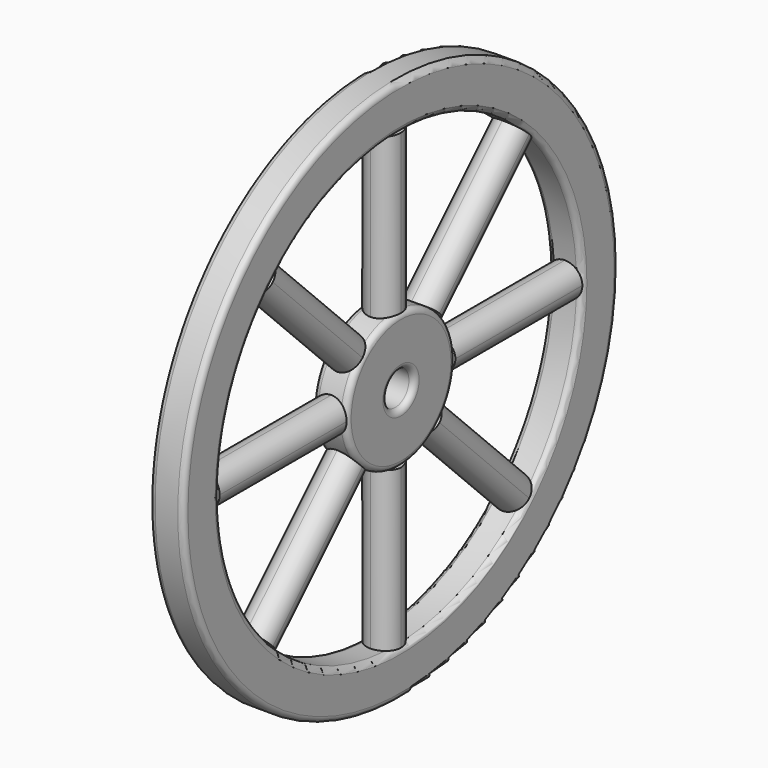
from build123d import *

# Parameters (mm, degrees)
F0_R          = 304.8
F0_R_2        = 254
F1_DEPTH      = 19.05
F2_R          = 76.2
F2_R_2        = 19.05
F3_DEPTH      = 19.05
F4_R          = 6.35
F4_2_R        = 6.35
F6_DEPTH      = 19.05
F7_T4_DEPTH   = 274.7542848295
F7_S5_R       = 76.2
F7_T6_DEPTH   = 140
F7_S7_R       = 254
F7_T8_DEPTH   = 140
F7_T12_DEPTH  = 274.7542848295
F7_S13_R      = 76.2
F7_T14_DEPTH  = 140
F7_S15_R      = 254
F7_T16_DEPTH  = 140
F7_T20_DEPTH  = 274.7542848295
F7_S21_R      = 76.2
F7_T22_DEPTH  = 140
F7_S23_R      = 254
F7_T24_DEPTH  = 140
F7_T28_DEPTH  = 274.7542848295
F7_S29_R      = 76.2
F7_T30_DEPTH  = 140
F7_S31_R      = 254
F7_T32_DEPTH  = 140
F7_T36_DEPTH  = 274.7542848295
F7_S37_R      = 76.2
F7_T38_DEPTH  = 149
F7_S39_R      = 254
F7_T40_DEPTH  = 149
F7_T44_DEPTH  = 274.7542848295
F7_S45_R      = 76.2
F7_T46_DEPTH  = 149
F7_S47_R      = 254
F7_T48_DEPTH  = 149
F7_T52_DEPTH  = 274.7542848295
F7_S53_R      = 76.2
F7_T54_DEPTH  = 149
F7_S55_R      = 254
F7_T56_DEPTH  = 149
F7_T60_DEPTH  = 274.7542848295
F7_S61_R      = 76.2
F7_T62_DEPTH  = 149
F7_S63_R      = 254
F7_T64_DEPTH  = 149
F7_T68_DEPTH  = 274.7542848295
F7_S69_R      = 76.2
F7_T70_DEPTH  = 140
F7_S71_R      = 254
F7_T72_DEPTH  = 140
F7_T76_DEPTH  = 274.7542848295
F7_S77_R      = 76.2
F7_T78_DEPTH  = 140
F7_S79_R      = 254
F7_T80_DEPTH  = 140
F7_T84_DEPTH  = 274.7542848295
F7_S85_R      = 76.2
F7_T86_DEPTH  = 140
F7_S87_R      = 254
F7_T88_DEPTH  = 140
F7_T92_DEPTH  = 274.7542848295
F7_S93_R      = 76.2
F7_T94_DEPTH  = 140
F7_S95_R      = 254
F7_T96_DEPTH  = 140
F7_T100_DEPTH = 274.7542848295
F7_S101_R     = 76.2
F7_T102_DEPTH = 149
F7_S103_R     = 254
F7_T104_DEPTH = 149
F7_T108_DEPTH = 274.7542848295
F7_S109_R     = 76.2
F7_T110_DEPTH = 149
F7_S111_R     = 254
F7_T112_DEPTH = 149
F7_T116_DEPTH = 274.7542848295
F7_S117_R     = 76.2
F7_T118_DEPTH = 149
F7_S119_R     = 254
F7_T120_DEPTH = 149
F7_T124_DEPTH = 274.7542848295
F7_S125_R     = 76.2
F7_T126_DEPTH = 149
F7_S127_R     = 254
F7_T128_DEPTH = 149
F7_T132_DEPTH = 274.7542848295
F7_S133_R     = 76.2
F7_T134_DEPTH = 140
F7_S135_R     = 254
F7_T136_DEPTH = 140
F7_T140_DEPTH = 274.7542848295
F7_S141_R     = 76.2
F7_T142_DEPTH = 140
F7_S143_R     = 254
F7_T144_DEPTH = 140
F7_T148_DEPTH = 274.7542848295
F7_S149_R     = 76.2
F7_T150_DEPTH = 140
F7_S151_R     = 254
F7_T152_DEPTH = 140
F7_T156_DEPTH = 274.7542848295
F7_S157_R     = 76.2
F7_T158_DEPTH = 140
F7_S159_R     = 254
F7_T160_DEPTH = 140
F7_T164_DEPTH = 274.7542848295
F7_S165_R     = 76.2
F7_T166_DEPTH = 149
F7_S167_R     = 254
F7_T168_DEPTH = 149
F7_T172_DEPTH = 274.7542848295
F7_S173_R     = 76.2
F7_T174_DEPTH = 149
F7_S175_R     = 254
F7_T176_DEPTH = 149
F7_T180_DEPTH = 274.7542848295
F7_S181_R     = 76.2
F7_T182_DEPTH = 149
F7_S183_R     = 254
F7_T184_DEPTH = 149
F7_T188_DEPTH = 274.7542848295
F7_S189_R     = 76.2
F7_T190_DEPTH = 149
F7_S191_R     = 254
F7_T192_DEPTH = 149
F7_T196_DEPTH = 274.7542848295
F7_S197_R     = 76.2
F7_T198_DEPTH = 140
F7_S199_R     = 254
F7_T200_DEPTH = 140
F7_T204_DEPTH = 274.7542848295
F7_S205_R     = 76.2
F7_T206_DEPTH = 140
F7_S207_R     = 254
F7_T208_DEPTH = 140
F7_T212_DEPTH = 274.7542848295
F7_S213_R     = 76.2
F7_T214_DEPTH = 140
F7_S215_R     = 254
F7_T216_DEPTH = 140
F7_T220_DEPTH = 274.7542848295
F7_S221_R     = 76.2
F7_T222_DEPTH = 140
F7_S223_R     = 254
F7_T224_DEPTH = 140
F7_T228_DEPTH = 274.7542848295
F7_S229_R     = 76.2
F7_T230_DEPTH = 149
F7_S231_R     = 254
F7_T232_DEPTH = 149
F7_T236_DEPTH = 274.7542848295
F7_S237_R     = 76.2
F7_T238_DEPTH = 149
F7_S239_R     = 254
F7_T240_DEPTH = 149
F7_T244_DEPTH = 274.7542848295
F7_S245_R     = 76.2
F7_T246_DEPTH = 149
F7_S247_R     = 254
F7_T248_DEPTH = 149
F7_T252_DEPTH = 274.7542848295
F7_S253_R     = 76.2
F7_T254_DEPTH = 149
F7_S255_R     = 254
F7_T256_DEPTH = 149


# Not quite as in the source:
# - a fillet or chamfer that OpenCascade refuses, or shapes differently, is made with other operations: its cross-section is extruded or revolved along the edge and cut away or added


with BuildPart() as f1:
    # F0 (on Right) → F1 (new body, symmetric)
    with BuildSketch(Plane.YZ):
        Circle(F0_R)
        Circle(F0_R_2, mode=Mode.SUBTRACT)
    extrude(amount=F1_DEPTH, both=True)

    # F4
    f4_edges = [f1.edges().sort_by_distance(p)[0] for p in [
        (19.05, -304.8, 0),
        (-19.05, -304.8, 0),
        (19.05, -254, 0),
        (-19.05, -254, 0),
    ]]
    fillet(f4_edges, radius=F4_R)



with BuildPart() as f3:
    # F2 (on Right) → F3 (new body, symmetric)
    with BuildSketch(Plane.YZ):
        Circle(F2_R)
        Circle(F2_R_2, mode=Mode.SUBTRACT)
    extrude(amount=F3_DEPTH, both=True)

    # F4#2
    f4_2_edges = [f3.edges().sort_by_distance(p)[0] for p in [
        (-19.05, -76.2, 0),
        (19.05, -76.2, 0),
        (19.05, -19.05, 0),
        (-19.05, -19.05, 0),
    ]]
    fillet(f4_2_edges, radius=F4_2_R)


with BuildPart() as f1_1:
    add(f1.part)

    add(f3.part)  # F6 merges F3
    # F5 (on Right) → F6 (join, symmetric)
    with BuildSketch(Plane.YZ):
        with BuildLine():
            Line((19.05, 73.7803327453), (19.05, 253.2846175748))
            ThreePointArc((19.05, 253.2846175748), (0, 254), (-19.05, 253.2846175748))
            Line((-19.05, 253.2846175748), (-19.05, 73.7803327453))
            ThreePointArc((-19.05, 73.7803327453), (0, 76.2), (19.05, 73.7803327453))
        make_face()
        with BuildLine():
            ThreePointArc((-65.640957784, 38.7001894208), (-53.8815367264, 53.8815367264), (-38.7001894208, 65.640957784))
            Line((-38.7001894208, 65.640957784), (-165.6288864758, 192.569654839))
            ThreePointArc((-165.6288864758, 192.569654839), (-179.6051224214, 179.6051224214), (-192.569654839, 165.6288864758))
            Line((-192.569654839, 165.6288864758), (-65.640957784, 38.7001894208))
        make_face()
        with BuildLine():
            ThreePointArc((-73.7803327453, -19.05), (-76.2, 0), (-73.7803327453, 19.05))
            Line((-73.7803327453, 19.05), (-253.2846175748, 19.05))
            ThreePointArc((-253.2846175748, 19.05), (-254, 0), (-253.2846175748, -19.05))
            Line((-253.2846175748, -19.05), (-73.7803327453, -19.05))
        make_face()
        with BuildLine():
            ThreePointArc((-38.7001894208, -65.640957784), (-53.8815367264, -53.8815367264), (-65.640957784, -38.7001894208))
            Line((-65.640957784, -38.7001894208), (-192.569654839, -165.6288864758))
            ThreePointArc((-192.569654839, -165.6288864758), (-179.6051224214, -179.6051224214), (-165.6288864758, -192.569654839))
            Line((-165.6288864758, -192.569654839), (-38.7001894208, -65.640957784))
        make_face()
        with BuildLine():
            ThreePointArc((19.05, -73.7803327453), (0, -76.2), (-19.05, -73.7803327453))
            Line((-19.05, -73.7803327453), (-19.05, -253.2846175748))
            ThreePointArc((-19.05, -253.2846175748), (0, -254), (19.05, -253.2846175748))
            Line((19.05, -253.2846175748), (19.05, -73.7803327453))
        make_face()
        with BuildLine():
            ThreePointArc((65.640957784, -38.7001894208), (53.8815367264, -53.8815367264), (38.7001894208, -65.640957784))
            Line((38.7001894208, -65.640957784), (165.6288864758, -192.569654839))
            ThreePointArc((165.6288864758, -192.569654839), (179.6051224214, -179.6051224214), (192.569654839, -165.6288864758))
            Line((192.569654839, -165.6288864758), (65.640957784, -38.7001894208))
        make_face()
        with BuildLine():
            ThreePointArc((73.7803327453, 19.05), (76.2, 0), (73.7803327453, -19.05))
            Line((73.7803327453, -19.05), (253.2846175748, -19.05))
            ThreePointArc((253.2846175748, -19.05), (254, 0), (253.2846175748, 19.05))
            Line((253.2846175748, 19.05), (73.7803327453, 19.05))
        make_face()
        with BuildLine():
            ThreePointArc((38.7001894208, 65.640957784), (53.8815367264, 53.8815367264), (65.640957784, 38.7001894208))
            Line((65.640957784, 38.7001894208), (192.569654839, 165.6288864758))
            ThreePointArc((192.569654839, 165.6288864758), (179.6051224214, 179.6051224214), (165.6288864758, 192.569654839))
            Line((165.6288864758, 192.569654839), (38.7001894208, 65.640957784))
        make_face()
    extrude(amount=F6_DEPTH, both=True)

    # F7: fillet of radius 19.05 on 32 edges, made by hand


with BuildPart() as f7_tool2:
    # F7_s3 → F7_t4 (new body)
    with BuildSketch(Plane.XY.offset(26.1553327453)):
        with BuildLine():
            ThreePointArc((19.05, 0), (13.4703841816, 13.4703841816), (0, 19.05))
            Line((0, 19.05), (19.05, 19.05))
            Line((19.05, 19.05), (19.05, 0))
        make_face()
    extrude(amount=F7_T4_DEPTH)

    # F7_s5 → F7_t6 (cut, symmetric)
    with BuildSketch(Plane.YZ.offset(9.5)):
        Circle(F7_S5_R)
    extrude(amount=F7_T6_DEPTH, both=True, mode=Mode.SUBTRACT)

    # F7_s7 → F7_t8 (intersect, symmetric)
    with BuildSketch(Plane.YZ.offset(9.5)):
        Circle(F7_S7_R)
    extrude(amount=F7_T8_DEPTH, both=True, mode=Mode.INTERSECT)


with BuildPart() as f1_2:
    add(f1_1.part)

    # F7_t1: cut F7_tool2
    add(f7_tool2.part, mode=Mode.SUBTRACT)


with BuildPart() as f7_tool10:
    # F7_s11 → F7_t12 (new body)
    with BuildSketch(Plane.XY.offset(300.9096175748)):
        with BuildLine():
            ThreePointArc((0, -19.05), (13.4703841816, -13.4703841816), (19.05, 0))
            Line((19.05, 0), (19.05, -19.05))
            Line((19.05, -19.05), (0, -19.05))
        make_face()
    extrude(amount=-F7_T12_DEPTH)

    # F7_s13 → F7_t14 (cut, symmetric)
    with BuildSketch(Plane.YZ.offset(9.5)):
        Circle(F7_S13_R)
    extrude(amount=F7_T14_DEPTH, both=True, mode=Mode.SUBTRACT)

    # F7_s15 → F7_t16 (intersect, symmetric)
    with BuildSketch(Plane.YZ.offset(9.5)):
        Circle(F7_S15_R)
    extrude(amount=F7_T16_DEPTH, both=True, mode=Mode.INTERSECT)


with BuildPart() as f1_3:
    add(f1_2.part)

    # F7_t9: cut F7_tool10
    add(f7_tool10.part, mode=Mode.SUBTRACT)


with BuildPart() as f7_tool18:
    # F7_s19 → F7_t20 (new body)
    with BuildSketch(Plane.XY.offset(300.9096175748)):
        with BuildLine():
            ThreePointArc((0, -19.05), (-13.4703841816, -13.4703841816), (-19.05, 0))
            Line((-19.05, 0), (-19.05, -19.05))
            Line((-19.05, -19.05), (0, -19.05))
        make_face()
    extrude(amount=-F7_T20_DEPTH)

    # F7_s21 → F7_t22 (cut, symmetric)
    with BuildSketch(Plane.YZ.offset(-9.5)):
        Circle(F7_S21_R)
    extrude(amount=F7_T22_DEPTH, both=True, mode=Mode.SUBTRACT)

    # F7_s23 → F7_t24 (intersect, symmetric)
    with BuildSketch(Plane.YZ.offset(-9.5)):
        Circle(F7_S23_R)
    extrude(amount=F7_T24_DEPTH, both=True, mode=Mode.INTERSECT)


with BuildPart() as f1_4:
    add(f1_3.part)

    # F7_t17: cut F7_tool18
    add(f7_tool18.part, mode=Mode.SUBTRACT)


with BuildPart() as f7_tool26:
    # F7_s27 → F7_t28 (new body)
    with BuildSketch(Plane.XY.offset(26.1553327453)):
        with BuildLine():
            ThreePointArc((0, 19.05), (-13.4703841816, 13.4703841816), (-19.05, 0))
            Line((-19.05, 0), (-19.05, 19.05))
            Line((-19.05, 19.05), (0, 19.05))
        make_face()
    extrude(amount=F7_T28_DEPTH)

    # F7_s29 → F7_t30 (cut, symmetric)
    with BuildSketch(Plane.YZ.offset(-9.5)):
        Circle(F7_S29_R)
    extrude(amount=F7_T30_DEPTH, both=True, mode=Mode.SUBTRACT)

    # F7_s31 → F7_t32 (intersect, symmetric)
    with BuildSketch(Plane.YZ.offset(-9.5)):
        Circle(F7_S31_R)
    extrude(amount=F7_T32_DEPTH, both=True, mode=Mode.INTERSECT)


with BuildPart() as f1_5:
    add(f1_4.part)

    # F7_t25: cut F7_tool26
    add(f7_tool26.part, mode=Mode.SUBTRACT)


with BuildPart() as f7_tool34:
    # F7_s35 → F7_t36 (new body)
    with BuildSketch(Plane(origin=(0, -18.4946131484, 18.4946131484), x_dir=(1, 0, 0), z_dir=(0, -0.7071067812, 0.7071067812))):
        with BuildLine():
            ThreePointArc((0, 19.05), (-13.4703841816, 13.4703841816), (-19.05, 0))
            Line((-19.05, 0), (-19.05, 19.05))
            Line((-19.05, 19.05), (0, 19.05))
        make_face()
    extrude(amount=F7_T36_DEPTH)

    # F7_s37 → F7_t38 (cut, symmetric)
    with BuildSketch(Plane.YZ.offset(-9.5)):
        Circle(F7_S37_R)
    extrude(amount=F7_T38_DEPTH, both=True, mode=Mode.SUBTRACT)

    # F7_s39 → F7_t40 (intersect, symmetric)
    with BuildSketch(Plane.YZ.offset(-9.5)):
        Circle(F7_S39_R)
    extrude(amount=F7_T40_DEPTH, both=True, mode=Mode.INTERSECT)


with BuildPart() as f1_6:
    add(f1_5.part)

    # F7_t33: cut F7_tool34
    add(f7_tool34.part, mode=Mode.SUBTRACT)


with BuildPart() as f7_tool42:
    # F7_s43 → F7_t44 (new body)
    with BuildSketch(Plane(origin=(0, -18.4946131484, 18.4946131484), x_dir=(1, 0, 0), z_dir=(0, -0.7071067812, 0.7071067812))):
        with BuildLine():
            ThreePointArc((19.05, 0), (13.4703841816, 13.4703841816), (0, 19.05))
            Line((0, 19.05), (19.05, 19.05))
            Line((19.05, 19.05), (19.05, 0))
        make_face()
    extrude(amount=F7_T44_DEPTH)

    # F7_s45 → F7_t46 (cut, symmetric)
    with BuildSketch(Plane.YZ.offset(9.5)):
        Circle(F7_S45_R)
    extrude(amount=F7_T46_DEPTH, both=True, mode=Mode.SUBTRACT)

    # F7_s47 → F7_t48 (intersect, symmetric)
    with BuildSketch(Plane.YZ.offset(9.5)):
        Circle(F7_S47_R)
    extrude(amount=F7_T48_DEPTH, both=True, mode=Mode.INTERSECT)


with BuildPart() as f1_7:
    add(f1_6.part)

    # F7_t41: cut F7_tool42
    add(f7_tool42.part, mode=Mode.SUBTRACT)


with BuildPart() as f7_tool50:
    # F7_s51 → F7_t52 (new body)
    with BuildSketch(Plane(origin=(0, -212.7752311114, 212.7752311114), x_dir=(1, 0, 0), z_dir=(0, 0.7071067812, -0.7071067812))):
        with BuildLine():
            ThreePointArc((0, 19.05), (-13.4703841816, 13.4703841816), (-19.05, 0))
            Line((-19.05, 0), (-19.05, 19.05))
            Line((-19.05, 19.05), (0, 19.05))
        make_face()
    extrude(amount=F7_T52_DEPTH)

    # F7_s53 → F7_t54 (cut, symmetric)
    with BuildSketch(Plane.YZ.offset(-9.5)):
        Circle(F7_S53_R)
    extrude(amount=F7_T54_DEPTH, both=True, mode=Mode.SUBTRACT)

    # F7_s55 → F7_t56 (intersect, symmetric)
    with BuildSketch(Plane.YZ.offset(-9.5)):
        Circle(F7_S55_R)
    extrude(amount=F7_T56_DEPTH, both=True, mode=Mode.INTERSECT)


with BuildPart() as f1_8:
    add(f1_7.part)

    # F7_t49: cut F7_tool50
    add(f7_tool50.part, mode=Mode.SUBTRACT)


with BuildPart() as f7_tool58:
    # F7_s59 → F7_t60 (new body)
    with BuildSketch(Plane(origin=(0, -212.7752311114, 212.7752311114), x_dir=(1, 0, 0), z_dir=(0, 0.7071067812, -0.7071067812))):
        with BuildLine():
            ThreePointArc((0, 19.05), (13.4703841816, 13.4703841816), (19.05, 0))
            Line((19.05, 0), (19.05, 19.05))
            Line((19.05, 19.05), (0, 19.05))
        make_face()
    extrude(amount=F7_T60_DEPTH)

    # F7_s61 → F7_t62 (cut, symmetric)
    with BuildSketch(Plane.YZ.offset(9.5)):
        Circle(F7_S61_R)
    extrude(amount=F7_T62_DEPTH, both=True, mode=Mode.SUBTRACT)

    # F7_s63 → F7_t64 (intersect, symmetric)
    with BuildSketch(Plane.YZ.offset(9.5)):
        Circle(F7_S63_R)
    extrude(amount=F7_T64_DEPTH, both=True, mode=Mode.INTERSECT)


with BuildPart() as f1_9:
    add(f1_8.part)

    # F7_t57: cut F7_tool58
    add(f7_tool58.part, mode=Mode.SUBTRACT)


with BuildPart() as f7_tool66:
    # F7_s67 → F7_t68 (new body)
    with BuildSketch(Plane.XZ.offset(26.1553327453)):
        with BuildLine():
            ThreePointArc((19.05, 0), (13.4703841816, 13.4703841816), (0, 19.05))
            Line((0, 19.05), (19.05, 19.05))
            Line((19.05, 19.05), (19.05, 0))
        make_face()
    extrude(amount=F7_T68_DEPTH)

    # F7_s69 → F7_t70 (cut, symmetric)
    with BuildSketch(Plane.YZ.offset(9.5)):
        Circle(F7_S69_R)
    extrude(amount=F7_T70_DEPTH, both=True, mode=Mode.SUBTRACT)

    # F7_s71 → F7_t72 (intersect, symmetric)
    with BuildSketch(Plane.YZ.offset(9.5)):
        Circle(F7_S71_R)
    extrude(amount=F7_T72_DEPTH, both=True, mode=Mode.INTERSECT)


with BuildPart() as f1_10:
    add(f1_9.part)

    # F7_t65: cut F7_tool66
    add(f7_tool66.part, mode=Mode.SUBTRACT)


with BuildPart() as f7_tool74:
    # F7_s75 → F7_t76 (new body)
    with BuildSketch(Plane.XZ.offset(26.1553327453)):
        with BuildLine():
            ThreePointArc((0, 19.05), (-13.4703841816, 13.4703841816), (-19.05, 0))
            Line((-19.05, 0), (-19.05, 19.05))
            Line((-19.05, 19.05), (0, 19.05))
        make_face()
    extrude(amount=F7_T76_DEPTH)

    # F7_s77 → F7_t78 (cut, symmetric)
    with BuildSketch(Plane.YZ.offset(-9.5)):
        Circle(F7_S77_R)
    extrude(amount=F7_T78_DEPTH, both=True, mode=Mode.SUBTRACT)

    # F7_s79 → F7_t80 (intersect, symmetric)
    with BuildSketch(Plane.YZ.offset(-9.5)):
        Circle(F7_S79_R)
    extrude(amount=F7_T80_DEPTH, both=True, mode=Mode.INTERSECT)


with BuildPart() as f1_11:
    add(f1_10.part)

    # F7_t73: cut F7_tool74
    add(f7_tool74.part, mode=Mode.SUBTRACT)


with BuildPart() as f7_tool82:
    # F7_s83 → F7_t84 (new body)
    with BuildSketch(Plane.XZ.offset(300.9096175748)):
        with BuildLine():
            ThreePointArc((0, -19.05), (-13.4703841816, -13.4703841816), (-19.05, 0))
            Line((-19.05, 0), (-19.05, -19.05))
            Line((-19.05, -19.05), (0, -19.05))
        make_face()
    extrude(amount=-F7_T84_DEPTH)

    # F7_s85 → F7_t86 (cut, symmetric)
    with BuildSketch(Plane.YZ.offset(-9.5)):
        Circle(F7_S85_R)
    extrude(amount=F7_T86_DEPTH, both=True, mode=Mode.SUBTRACT)

    # F7_s87 → F7_t88 (intersect, symmetric)
    with BuildSketch(Plane.YZ.offset(-9.5)):
        Circle(F7_S87_R)
    extrude(amount=F7_T88_DEPTH, both=True, mode=Mode.INTERSECT)


with BuildPart() as f1_12:
    add(f1_11.part)

    # F7_t81: cut F7_tool82
    add(f7_tool82.part, mode=Mode.SUBTRACT)


with BuildPart() as f7_tool90:
    # F7_s91 → F7_t92 (new body)
    with BuildSketch(Plane.XZ.offset(300.9096175748)):
        with BuildLine():
            ThreePointArc((0, -19.05), (13.4703841816, -13.4703841816), (19.05, 0))
            Line((19.05, 0), (19.05, -19.05))
            Line((19.05, -19.05), (0, -19.05))
        make_face()
    extrude(amount=-F7_T92_DEPTH)

    # F7_s93 → F7_t94 (cut, symmetric)
    with BuildSketch(Plane.YZ.offset(9.5)):
        Circle(F7_S93_R)
    extrude(amount=F7_T94_DEPTH, both=True, mode=Mode.SUBTRACT)

    # F7_s95 → F7_t96 (intersect, symmetric)
    with BuildSketch(Plane.YZ.offset(9.5)):
        Circle(F7_S95_R)
    extrude(amount=F7_T96_DEPTH, both=True, mode=Mode.INTERSECT)


with BuildPart() as f1_13:
    add(f1_12.part)

    # F7_t89: cut F7_tool90
    add(f7_tool90.part, mode=Mode.SUBTRACT)


with BuildPart() as f7_tool98:
    # F7_s99 → F7_t100 (new body)
    with BuildSketch(Plane(origin=(0, -18.4946131484, -18.4946131484), x_dir=(1, 0, 0), z_dir=(0, -0.7071067812, -0.7071067812))):
        with BuildLine():
            ThreePointArc((19.05, 0), (13.4703841816, 13.4703841816), (0, 19.05))
            Line((0, 19.05), (19.05, 19.05))
            Line((19.05, 19.05), (19.05, 0))
        make_face()
    extrude(amount=F7_T100_DEPTH)

    # F7_s101 → F7_t102 (cut, symmetric)
    with BuildSketch(Plane.YZ.offset(9.5)):
        Circle(F7_S101_R)
    extrude(amount=F7_T102_DEPTH, both=True, mode=Mode.SUBTRACT)

    # F7_s103 → F7_t104 (intersect, symmetric)
    with BuildSketch(Plane.YZ.offset(9.5)):
        Circle(F7_S103_R)
    extrude(amount=F7_T104_DEPTH, both=True, mode=Mode.INTERSECT)


with BuildPart() as f1_14:
    add(f1_13.part)

    # F7_t97: cut F7_tool98
    add(f7_tool98.part, mode=Mode.SUBTRACT)


with BuildPart() as f7_tool106:
    # F7_s107 → F7_t108 (new body)
    with BuildSketch(Plane(origin=(0, -212.7752311114, -212.7752311114), x_dir=(1, 0, 0), z_dir=(0, 0.7071067812, 0.7071067812))):
        with BuildLine():
            ThreePointArc((0, 19.05), (13.4703841816, 13.4703841816), (19.05, 0))
            Line((19.05, 0), (19.05, 19.05))
            Line((19.05, 19.05), (0, 19.05))
        make_face()
    extrude(amount=F7_T108_DEPTH)

    # F7_s109 → F7_t110 (cut, symmetric)
    with BuildSketch(Plane.YZ.offset(9.5)):
        Circle(F7_S109_R)
    extrude(amount=F7_T110_DEPTH, both=True, mode=Mode.SUBTRACT)

    # F7_s111 → F7_t112 (intersect, symmetric)
    with BuildSketch(Plane.YZ.offset(9.5)):
        Circle(F7_S111_R)
    extrude(amount=F7_T112_DEPTH, both=True, mode=Mode.INTERSECT)


with BuildPart() as f1_15:
    add(f1_14.part)

    # F7_t105: cut F7_tool106
    add(f7_tool106.part, mode=Mode.SUBTRACT)


with BuildPart() as f7_tool114:
    # F7_s115 → F7_t116 (new body)
    with BuildSketch(Plane(origin=(0, -18.4946131484, -18.4946131484), x_dir=(1, 0, 0), z_dir=(0, -0.7071067812, -0.7071067812))):
        with BuildLine():
            ThreePointArc((0, 19.05), (-13.4703841816, 13.4703841816), (-19.05, 0))
            Line((-19.05, 0), (-19.05, 19.05))
            Line((-19.05, 19.05), (0, 19.05))
        make_face()
    extrude(amount=F7_T116_DEPTH)

    # F7_s117 → F7_t118 (cut, symmetric)
    with BuildSketch(Plane.YZ.offset(-9.5)):
        Circle(F7_S117_R)
    extrude(amount=F7_T118_DEPTH, both=True, mode=Mode.SUBTRACT)

    # F7_s119 → F7_t120 (intersect, symmetric)
    with BuildSketch(Plane.YZ.offset(-9.5)):
        Circle(F7_S119_R)
    extrude(amount=F7_T120_DEPTH, both=True, mode=Mode.INTERSECT)


with BuildPart() as f1_16:
    add(f1_15.part)

    # F7_t113: cut F7_tool114
    add(f7_tool114.part, mode=Mode.SUBTRACT)


with BuildPart() as f7_tool122:
    # F7_s123 → F7_t124 (new body)
    with BuildSketch(Plane(origin=(0, -212.7752311114, -212.7752311114), x_dir=(1, 0, 0), z_dir=(0, 0.7071067812, 0.7071067812))):
        with BuildLine():
            ThreePointArc((0, 19.05), (-13.4703841816, 13.4703841816), (-19.05, 0))
            Line((-19.05, 0), (-19.05, 19.05))
            Line((-19.05, 19.05), (0, 19.05))
        make_face()
    extrude(amount=F7_T124_DEPTH)

    # F7_s125 → F7_t126 (cut, symmetric)
    with BuildSketch(Plane.YZ.offset(-9.5)):
        Circle(F7_S125_R)
    extrude(amount=F7_T126_DEPTH, both=True, mode=Mode.SUBTRACT)

    # F7_s127 → F7_t128 (intersect, symmetric)
    with BuildSketch(Plane.YZ.offset(-9.5)):
        Circle(F7_S127_R)
    extrude(amount=F7_T128_DEPTH, both=True, mode=Mode.INTERSECT)


with BuildPart() as f1_17:
    add(f1_16.part)

    # F7_t121: cut F7_tool122
    add(f7_tool122.part, mode=Mode.SUBTRACT)


with BuildPart() as f7_tool130:
    # F7_s131 → F7_t132 (new body)
    with BuildSketch(Plane.XY.offset(-26.1553327453)):
        with BuildLine():
            ThreePointArc((0, -19.05), (-13.4703841816, -13.4703841816), (-19.05, 0))
            Line((-19.05, 0), (-19.05, -19.05))
            Line((-19.05, -19.05), (0, -19.05))
        make_face()
    extrude(amount=-F7_T132_DEPTH)

    # F7_s133 → F7_t134 (cut, symmetric)
    with BuildSketch(Plane.YZ.offset(-9.5)):
        Circle(F7_S133_R)
    extrude(amount=F7_T134_DEPTH, both=True, mode=Mode.SUBTRACT)

    # F7_s135 → F7_t136 (intersect, symmetric)
    with BuildSketch(Plane.YZ.offset(-9.5)):
        Circle(F7_S135_R)
    extrude(amount=F7_T136_DEPTH, both=True, mode=Mode.INTERSECT)


with BuildPart() as f1_18:
    add(f1_17.part)

    # F7_t129: cut F7_tool130
    add(f7_tool130.part, mode=Mode.SUBTRACT)


with BuildPart() as f7_tool138:
    # F7_s139 → F7_t140 (new body)
    with BuildSketch(Plane.XY.offset(-26.1553327453)):
        with BuildLine():
            ThreePointArc((19.05, 0), (13.4703841816, -13.4703841816), (0, -19.05))
            Line((0, -19.05), (19.05, -19.05))
            Line((19.05, -19.05), (19.05, 0))
        make_face()
    extrude(amount=-F7_T140_DEPTH)

    # F7_s141 → F7_t142 (cut, symmetric)
    with BuildSketch(Plane.YZ.offset(9.5)):
        Circle(F7_S141_R)
    extrude(amount=F7_T142_DEPTH, both=True, mode=Mode.SUBTRACT)

    # F7_s143 → F7_t144 (intersect, symmetric)
    with BuildSketch(Plane.YZ.offset(9.5)):
        Circle(F7_S143_R)
    extrude(amount=F7_T144_DEPTH, both=True, mode=Mode.INTERSECT)


with BuildPart() as f1_19:
    add(f1_18.part)

    # F7_t137: cut F7_tool138
    add(f7_tool138.part, mode=Mode.SUBTRACT)


with BuildPart() as f7_tool146:
    # F7_s147 → F7_t148 (new body)
    with BuildSketch(Plane.XY.offset(-300.9096175748)):
        with BuildLine():
            ThreePointArc((0, 19.05), (13.4703841816, 13.4703841816), (19.05, 0))
            Line((19.05, 0), (19.05, 19.05))
            Line((19.05, 19.05), (0, 19.05))
        make_face()
    extrude(amount=F7_T148_DEPTH)

    # F7_s149 → F7_t150 (cut, symmetric)
    with BuildSketch(Plane.YZ.offset(9.5)):
        Circle(F7_S149_R)
    extrude(amount=F7_T150_DEPTH, both=True, mode=Mode.SUBTRACT)

    # F7_s151 → F7_t152 (intersect, symmetric)
    with BuildSketch(Plane.YZ.offset(9.5)):
        Circle(F7_S151_R)
    extrude(amount=F7_T152_DEPTH, both=True, mode=Mode.INTERSECT)


with BuildPart() as f1_20:
    add(f1_19.part)

    # F7_t145: cut F7_tool146
    add(f7_tool146.part, mode=Mode.SUBTRACT)


with BuildPart() as f7_tool154:
    # F7_s155 → F7_t156 (new body)
    with BuildSketch(Plane.XY.offset(-300.9096175748)):
        with BuildLine():
            ThreePointArc((0, 19.05), (-13.4703841816, 13.4703841816), (-19.05, 0))
            Line((-19.05, 0), (-19.05, 19.05))
            Line((-19.05, 19.05), (0, 19.05))
        make_face()
    extrude(amount=F7_T156_DEPTH)

    # F7_s157 → F7_t158 (cut, symmetric)
    with BuildSketch(Plane.YZ.offset(-9.5)):
        Circle(F7_S157_R)
    extrude(amount=F7_T158_DEPTH, both=True, mode=Mode.SUBTRACT)

    # F7_s159 → F7_t160 (intersect, symmetric)
    with BuildSketch(Plane.YZ.offset(-9.5)):
        Circle(F7_S159_R)
    extrude(amount=F7_T160_DEPTH, both=True, mode=Mode.INTERSECT)


with BuildPart() as f1_21:
    add(f1_20.part)

    # F7_t153: cut F7_tool154
    add(f7_tool154.part, mode=Mode.SUBTRACT)


with BuildPart() as f7_tool162:
    # F7_s163 → F7_t164 (new body)
    with BuildSketch(Plane(origin=(0, 18.4946131484, -18.4946131484), x_dir=(1, 0, 0), z_dir=(0, 0.7071067812, -0.7071067812))):
        with BuildLine():
            ThreePointArc((0, 19.05), (-13.4703841816, 13.4703841816), (-19.05, 0))
            Line((-19.05, 0), (-19.05, 19.05))
            Line((-19.05, 19.05), (0, 19.05))
        make_face()
    extrude(amount=F7_T164_DEPTH)

    # F7_s165 → F7_t166 (cut, symmetric)
    with BuildSketch(Plane.YZ.offset(-9.5)):
        Circle(F7_S165_R)
    extrude(amount=F7_T166_DEPTH, both=True, mode=Mode.SUBTRACT)

    # F7_s167 → F7_t168 (intersect, symmetric)
    with BuildSketch(Plane.YZ.offset(-9.5)):
        Circle(F7_S167_R)
    extrude(amount=F7_T168_DEPTH, both=True, mode=Mode.INTERSECT)


with BuildPart() as f1_22:
    add(f1_21.part)

    # F7_t161: cut F7_tool162
    add(f7_tool162.part, mode=Mode.SUBTRACT)


with BuildPart() as f7_tool170:
    # F7_s171 → F7_t172 (new body)
    with BuildSketch(Plane(origin=(0, 212.7752311114, -212.7752311114), x_dir=(1, 0, 0), z_dir=(0, -0.7071067812, 0.7071067812))):
        with BuildLine():
            ThreePointArc((0, 19.05), (-13.4703841816, 13.4703841816), (-19.05, 0))
            Line((-19.05, 0), (-19.05, 19.05))
            Line((-19.05, 19.05), (0, 19.05))
        make_face()
    extrude(amount=F7_T172_DEPTH)

    # F7_s173 → F7_t174 (cut, symmetric)
    with BuildSketch(Plane.YZ.offset(-9.5)):
        Circle(F7_S173_R)
    extrude(amount=F7_T174_DEPTH, both=True, mode=Mode.SUBTRACT)

    # F7_s175 → F7_t176 (intersect, symmetric)
    with BuildSketch(Plane.YZ.offset(-9.5)):
        Circle(F7_S175_R)
    extrude(amount=F7_T176_DEPTH, both=True, mode=Mode.INTERSECT)


with BuildPart() as f1_23:
    add(f1_22.part)

    # F7_t169: cut F7_tool170
    add(f7_tool170.part, mode=Mode.SUBTRACT)


with BuildPart() as f7_tool178:
    # F7_s179 → F7_t180 (new body)
    with BuildSketch(Plane(origin=(0, 18.4946131484, -18.4946131484), x_dir=(1, 0, 0), z_dir=(0, 0.7071067812, -0.7071067812))):
        with BuildLine():
            ThreePointArc((19.05, 0), (13.4703841816, 13.4703841816), (0, 19.05))
            Line((0, 19.05), (19.05, 19.05))
            Line((19.05, 19.05), (19.05, 0))
        make_face()
    extrude(amount=F7_T180_DEPTH)

    # F7_s181 → F7_t182 (cut, symmetric)
    with BuildSketch(Plane.YZ.offset(9.5)):
        Circle(F7_S181_R)
    extrude(amount=F7_T182_DEPTH, both=True, mode=Mode.SUBTRACT)

    # F7_s183 → F7_t184 (intersect, symmetric)
    with BuildSketch(Plane.YZ.offset(9.5)):
        Circle(F7_S183_R)
    extrude(amount=F7_T184_DEPTH, both=True, mode=Mode.INTERSECT)


with BuildPart() as f1_24:
    add(f1_23.part)

    # F7_t177: cut F7_tool178
    add(f7_tool178.part, mode=Mode.SUBTRACT)


with BuildPart() as f7_tool186:
    # F7_s187 → F7_t188 (new body)
    with BuildSketch(Plane(origin=(0, 212.7752311114, -212.7752311114), x_dir=(1, 0, 0), z_dir=(0, -0.7071067812, 0.7071067812))):
        with BuildLine():
            ThreePointArc((0, 19.05), (13.4703841816, 13.4703841816), (19.05, 0))
            Line((19.05, 0), (19.05, 19.05))
            Line((19.05, 19.05), (0, 19.05))
        make_face()
    extrude(amount=F7_T188_DEPTH)

    # F7_s189 → F7_t190 (cut, symmetric)
    with BuildSketch(Plane.YZ.offset(9.5)):
        Circle(F7_S189_R)
    extrude(amount=F7_T190_DEPTH, both=True, mode=Mode.SUBTRACT)

    # F7_s191 → F7_t192 (intersect, symmetric)
    with BuildSketch(Plane.YZ.offset(9.5)):
        Circle(F7_S191_R)
    extrude(amount=F7_T192_DEPTH, both=True, mode=Mode.INTERSECT)


with BuildPart() as f1_25:
    add(f1_24.part)

    # F7_t185: cut F7_tool186
    add(f7_tool186.part, mode=Mode.SUBTRACT)


with BuildPart() as f7_tool194:
    # F7_s195 → F7_t196 (new body)
    with BuildSketch(Plane.XZ.offset(-300.9096175748)):
        with BuildLine():
            ThreePointArc((0, 19.05), (13.4703841816, 13.4703841816), (19.05, 0))
            Line((19.05, 0), (19.05, 19.05))
            Line((19.05, 19.05), (0, 19.05))
        make_face()
    extrude(amount=F7_T196_DEPTH)

    # F7_s197 → F7_t198 (cut, symmetric)
    with BuildSketch(Plane.YZ.offset(9.5)):
        Circle(F7_S197_R)
    extrude(amount=F7_T198_DEPTH, both=True, mode=Mode.SUBTRACT)

    # F7_s199 → F7_t200 (intersect, symmetric)
    with BuildSketch(Plane.YZ.offset(9.5)):
        Circle(F7_S199_R)
    extrude(amount=F7_T200_DEPTH, both=True, mode=Mode.INTERSECT)


with BuildPart() as f1_26:
    add(f1_25.part)

    # F7_t193: cut F7_tool194
    add(f7_tool194.part, mode=Mode.SUBTRACT)


with BuildPart() as f7_tool202:
    # F7_s203 → F7_t204 (new body)
    with BuildSketch(Plane.XZ.offset(-26.1553327453)):
        with BuildLine():
            ThreePointArc((19.05, 0), (13.4703841816, -13.4703841816), (0, -19.05))
            Line((0, -19.05), (19.05, -19.05))
            Line((19.05, -19.05), (19.05, 0))
        make_face()
    extrude(amount=-F7_T204_DEPTH)

    # F7_s205 → F7_t206 (cut, symmetric)
    with BuildSketch(Plane.YZ.offset(9.5)):
        Circle(F7_S205_R)
    extrude(amount=F7_T206_DEPTH, both=True, mode=Mode.SUBTRACT)

    # F7_s207 → F7_t208 (intersect, symmetric)
    with BuildSketch(Plane.YZ.offset(9.5)):
        Circle(F7_S207_R)
    extrude(amount=F7_T208_DEPTH, both=True, mode=Mode.INTERSECT)


with BuildPart() as f1_27:
    add(f1_26.part)

    # F7_t201: cut F7_tool202
    add(f7_tool202.part, mode=Mode.SUBTRACT)


with BuildPart() as f7_tool210:
    # F7_s211 → F7_t212 (new body)
    with BuildSketch(Plane.XZ.offset(-300.9096175748)):
        with BuildLine():
            ThreePointArc((0, 19.05), (-13.4703841816, 13.4703841816), (-19.05, 0))
            Line((-19.05, 0), (-19.05, 19.05))
            Line((-19.05, 19.05), (0, 19.05))
        make_face()
    extrude(amount=F7_T212_DEPTH)

    # F7_s213 → F7_t214 (cut, symmetric)
    with BuildSketch(Plane.YZ.offset(-9.5)):
        Circle(F7_S213_R)
    extrude(amount=F7_T214_DEPTH, both=True, mode=Mode.SUBTRACT)

    # F7_s215 → F7_t216 (intersect, symmetric)
    with BuildSketch(Plane.YZ.offset(-9.5)):
        Circle(F7_S215_R)
    extrude(amount=F7_T216_DEPTH, both=True, mode=Mode.INTERSECT)


with BuildPart() as f1_28:
    add(f1_27.part)

    # F7_t209: cut F7_tool210
    add(f7_tool210.part, mode=Mode.SUBTRACT)


with BuildPart() as f7_tool218:
    # F7_s219 → F7_t220 (new body)
    with BuildSketch(Plane.XZ.offset(-26.1553327453)):
        with BuildLine():
            ThreePointArc((-19.05, 0), (-13.4703841816, -13.4703841816), (0, -19.05))
            Line((0, -19.05), (-19.05, -19.05))
            Line((-19.05, -19.05), (-19.05, 0))
        make_face()
    extrude(amount=-F7_T220_DEPTH)

    # F7_s221 → F7_t222 (cut, symmetric)
    with BuildSketch(Plane.YZ.offset(-9.5)):
        Circle(F7_S221_R)
    extrude(amount=F7_T222_DEPTH, both=True, mode=Mode.SUBTRACT)

    # F7_s223 → F7_t224 (intersect, symmetric)
    with BuildSketch(Plane.YZ.offset(-9.5)):
        Circle(F7_S223_R)
    extrude(amount=F7_T224_DEPTH, both=True, mode=Mode.INTERSECT)


with BuildPart() as f1_29:
    add(f1_28.part)

    # F7_t217: cut F7_tool218
    add(f7_tool218.part, mode=Mode.SUBTRACT)


with BuildPart() as f7_tool226:
    # F7_s227 → F7_t228 (new body)
    with BuildSketch(Plane(origin=(0, 212.7752311114, 212.7752311114), x_dir=(1, 0, 0), z_dir=(0, -0.7071067812, -0.7071067812))):
        with BuildLine():
            ThreePointArc((-19.05, 0), (-13.4703841816, 13.4703841816), (0, 19.05))
            Line((0, 19.05), (-19.05, 19.05))
            Line((-19.05, 19.05), (-19.05, 0))
        make_face()
    extrude(amount=F7_T228_DEPTH)

    # F7_s229 → F7_t230 (cut, symmetric)
    with BuildSketch(Plane.YZ.offset(-9.5)):
        Circle(F7_S229_R)
    extrude(amount=F7_T230_DEPTH, both=True, mode=Mode.SUBTRACT)

    # F7_s231 → F7_t232 (intersect, symmetric)
    with BuildSketch(Plane.YZ.offset(-9.5)):
        Circle(F7_S231_R)
    extrude(amount=F7_T232_DEPTH, both=True, mode=Mode.INTERSECT)


with BuildPart() as f1_30:
    add(f1_29.part)

    # F7_t225: cut F7_tool226
    add(f7_tool226.part, mode=Mode.SUBTRACT)


with BuildPart() as f7_tool234:
    # F7_s235 → F7_t236 (new body)
    with BuildSketch(Plane(origin=(0, 18.4946131484, 18.4946131484), x_dir=(1, 0, 0), z_dir=(0, 0.7071067812, 0.7071067812))):
        with BuildLine():
            ThreePointArc((0, 19.05), (-13.4703841816, 13.4703841816), (-19.05, 0))
            Line((-19.05, 0), (-19.05, 19.05))
            Line((-19.05, 19.05), (0, 19.05))
        make_face()
    extrude(amount=F7_T236_DEPTH)

    # F7_s237 → F7_t238 (cut, symmetric)
    with BuildSketch(Plane.YZ.offset(-9.5)):
        Circle(F7_S237_R)
    extrude(amount=F7_T238_DEPTH, both=True, mode=Mode.SUBTRACT)

    # F7_s239 → F7_t240 (intersect, symmetric)
    with BuildSketch(Plane.YZ.offset(-9.5)):
        Circle(F7_S239_R)
    extrude(amount=F7_T240_DEPTH, both=True, mode=Mode.INTERSECT)


with BuildPart() as f1_31:
    add(f1_30.part)

    # F7_t233: cut F7_tool234
    add(f7_tool234.part, mode=Mode.SUBTRACT)


with BuildPart() as f7_tool242:
    # F7_s243 → F7_t244 (new body)
    with BuildSketch(Plane(origin=(0, 18.4946131484, 18.4946131484), x_dir=(1, 0, 0), z_dir=(0, 0.7071067812, 0.7071067812))):
        with BuildLine():
            ThreePointArc((0, 19.05), (13.4703841816, 13.4703841816), (19.05, 0))
            Line((19.05, 0), (19.05, 19.05))
            Line((19.05, 19.05), (0, 19.05))
        make_face()
    extrude(amount=F7_T244_DEPTH)

    # F7_s245 → F7_t246 (cut, symmetric)
    with BuildSketch(Plane.YZ.offset(9.5)):
        Circle(F7_S245_R)
    extrude(amount=F7_T246_DEPTH, both=True, mode=Mode.SUBTRACT)

    # F7_s247 → F7_t248 (intersect, symmetric)
    with BuildSketch(Plane.YZ.offset(9.5)):
        Circle(F7_S247_R)
    extrude(amount=F7_T248_DEPTH, both=True, mode=Mode.INTERSECT)


with BuildPart() as f1_32:
    add(f1_31.part)

    # F7_t241: cut F7_tool242
    add(f7_tool242.part, mode=Mode.SUBTRACT)


with BuildPart() as f7_tool250:
    # F7_s251 → F7_t252 (new body)
    with BuildSketch(Plane(origin=(0, 212.7752311114, 212.7752311114), x_dir=(1, 0, 0), z_dir=(0, -0.7071067812, -0.7071067812))):
        with BuildLine():
            ThreePointArc((19.05, 0), (13.4703841816, 13.4703841816), (0, 19.05))
            Line((0, 19.05), (19.05, 19.05))
            Line((19.05, 19.05), (19.05, 0))
        make_face()
    extrude(amount=F7_T252_DEPTH)

    # F7_s253 → F7_t254 (cut, symmetric)
    with BuildSketch(Plane.YZ.offset(9.5)):
        Circle(F7_S253_R)
    extrude(amount=F7_T254_DEPTH, both=True, mode=Mode.SUBTRACT)

    # F7_s255 → F7_t256 (intersect, symmetric)
    with BuildSketch(Plane.YZ.offset(9.5)):
        Circle(F7_S255_R)
    extrude(amount=F7_T256_DEPTH, both=True, mode=Mode.INTERSECT)


with BuildPart() as f1_33:
    add(f1_32.part)

    # F7_t249: cut F7_tool250
    add(f7_tool250.part, mode=Mode.SUBTRACT)


solid = f1_33.part
